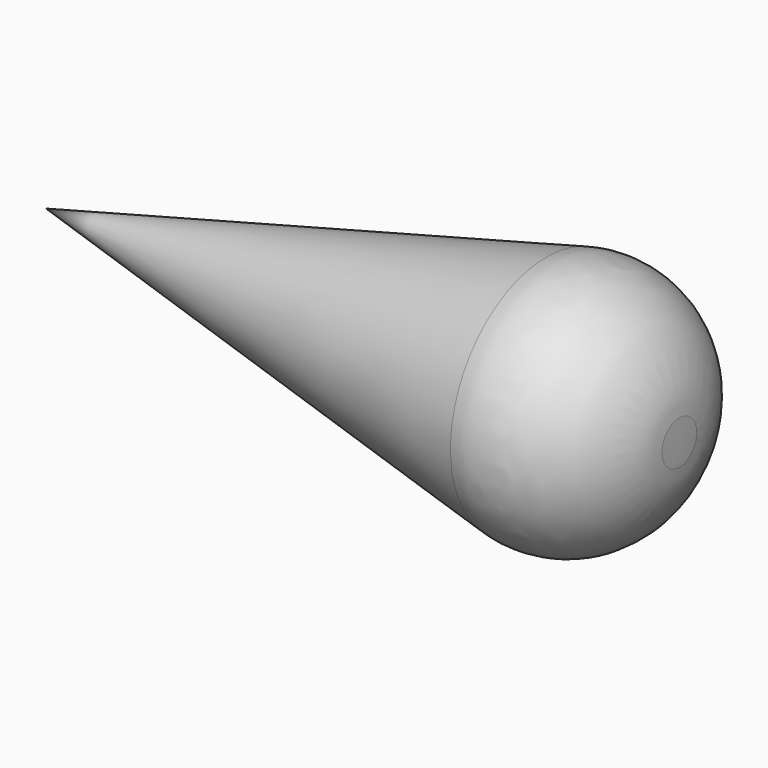
from build123d import *

# Parameters (mm, degrees)
F2_R = 17.6175907834


# Not quite as in the source:
# - a feature names something its author has since deleted; it is built from what else it names


with BuildPart() as f1:
    # F0 (on Top) → F1 (revolve)
    with BuildSketch(Plane.XY):
        with BuildLine():
            ThreePointArc((38.2172784488, 0), (36.9591747663, 12.0864529425), (33.2388062377, 23.654686499))
            Line((33.2388062377, 23.654686499), (-65.3415024281, 0))
            Line((-65.3415024281, 0), (38.2172784488, 0))
        make_face()
    revolve(axis=Axis((-7.6676234603, 0, 0), (1, 0, 0)))

    # F2
    f2_edges = [f1.edges().sort_by_distance(p)[0] for p in [
        (33.238806, -23.654686, 0),
    ]]
    fillet(f2_edges, radius=F2_R)


solid = f1.part
